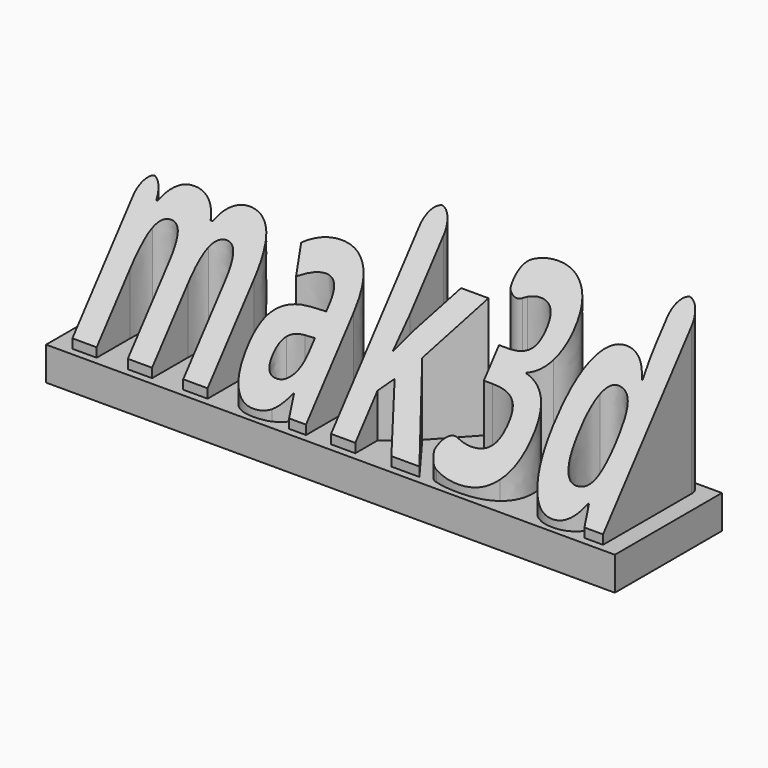
from build123d import *

# Parameters (mm, degrees)
F0_W         = 100
F0_H         = 20
F1_DEPTH     = 30
F4_DEPTH     = 15
F3_W         = 100
F3_H         = 20
F5_DEPTH     = 25
F6_DEPTH     = 200
F7_T4_DEPTH  = 29.5243209298
F7_T9_DEPTH  = 29.5243209298
F7_T14_DEPTH = 29.5243209298
F7_T19_DEPTH = 29.5243209298
F7_T24_DEPTH = 23.0076746252
F7_T29_DEPTH = 21.7768646713
F7_T34_DEPTH = 22.6661302513
F7_T39_DEPTH = 27.5964135534
F7_T44_DEPTH = 6.1840354013
F7_T49_DEPTH = 13.2594596433


# Not quite as in the source:
# - a fillet or chamfer that OpenCascade refuses, or shapes differently, is made with other operations: its cross-section is extruded or revolved along the edge and cut away or added


with BuildPart() as f1:
    # F0 (on Top) → F1 (new body)
    with BuildSketch(Plane.XY):
        with Locations((-50, 10)):
            Rectangle(F0_W, F0_H)
    extrude(amount=F1_DEPTH)

    # F4 (cut): a face of the model
    f4_faces = [f1.faces().sort_by_distance(p)[0] for p in [
        (0, 10, 15),
    ]]
    extrude(f4_faces, amount=-F4_DEPTH, mode=Mode.SUBTRACT)

    # F3 (on face) → F5 (cut)
    with BuildSketch(Plane.XY.offset(30)):
        with Locations((-50, 10)):
            Rectangle(F3_W, F3_H)
        with BuildLine():
            Line((-85.037182828, 7.7762018089), (-85.037182828, 1.100566471))
            Line((-85.037182828, 1.100566471), (-88.6663217196, 1.100566471))
            Line((-88.6663217196, 1.100566471), (-88.6663217196, 8.8729405296))
            add(Edge.make_bspline(
                [(-88.6663217196, 8.8729405296), (-88.6663217196, 10.3124101004), (-89.1480489702, 11.0321448859)],
                knots=[0, 0, 0, 1, 1, 1], degree=2))
            add(Edge.make_bspline(
                [(-89.1480489702, 11.0321448859), (-89.6297762207, 11.7518796713), (-90.6655850125, 11.7518796713)],
                knots=[0, 0, 0, 1, 1, 1], degree=2))
            add(Edge.make_bspline(
                [(-90.6655850125, 11.7518796713), (-92.0593571367, 11.7518796713), (-92.689601089, 10.7274952413)],
                knots=[0, 0, 0, 1, 1, 1], degree=2))
            add(Edge.make_bspline(
                [(-92.689601089, 10.7274952413), (-93.3198450413, 9.7031108112), (-93.3198450413, 7.3611166681)],
                knots=[0, 0, 0, 1, 1, 1], degree=2))
            Line((-93.3198450413, 7.3611166681), (-93.3198450413, 1.100566471))
            Line((-93.3198450413, 1.100566471), (-96.9489839329, 1.100566471))
            Line((-96.9489839329, 1.100566471), (-96.9489839329, 14.4061397001))
            Line((-96.9489839329, 14.4061397001), (-94.1766721668, 14.4061397001))
            Line((-94.1766721668, 14.4061397001), (-93.6892327354, 12.7039098108))
            Line((-93.6892327354, 12.7039098108), (-93.4874023458, 12.7039098108))
            add(Edge.make_bspline(
                [(-93.4874023458, 12.7039098108), (-92.9504573472, 13.6216668652), (-91.9394013391, 14.1376672008)],
                knots=[0, 0, 0, 1, 1, 1], degree=2))
            add(Edge.make_bspline(
                [(-91.9394013391, 14.1376672008), (-90.928345331, 14.6536675364), (-89.6183518591, 14.6536675364)],
                knots=[0, 0, 0, 1, 1, 1], degree=2))
            add(Edge.make_bspline(
                [(-89.6183518591, 14.6536675364), (-86.6327853417, 14.6536675364), (-85.5703197061, 12.7039098108)],
                knots=[0, 0, 0, 1, 1, 1], degree=2))
            Line((-85.5703197061, 12.7039098108), (-85.2504375792, 12.7039098108))
            add(Edge.make_bspline(
                [(-85.2504375792, 12.7039098108), (-84.7134925806, 13.6330912269), (-83.6738756683, 14.1433793816)],
                knots=[0, 0, 0, 1, 1, 1], degree=2))
            add(Edge.make_bspline(
                [(-83.6738756683, 14.1433793816), (-82.634258756, 14.6536675364), (-81.3242652841, 14.6536675364)],
                knots=[0, 0, 0, 1, 1, 1], degree=2))
            add(Edge.make_bspline(
                [(-81.3242652841, 14.6536675364), (-79.0622416727, 14.6536675364), (-77.9026689628, 13.4940948265)],
                knots=[0, 0, 0, 1, 1, 1], degree=2))
            add(Edge.make_bspline(
                [(-77.9026689628, 13.4940948265), (-76.743096253, 12.3345221167), (-76.743096253, 9.7754651018)],
                knots=[0, 0, 0, 1, 1, 1], degree=2))
            Line((-76.743096253, 9.7754651018), (-76.743096253, 1.100566471))
            Line((-76.743096253, 1.100566471), (-80.3836595063, 1.100566471))
            Line((-80.3836595063, 1.100566471), (-80.3836595063, 8.8729405296))
            add(Edge.make_bspline(
                [(-80.3836595063, 8.8729405296), (-80.3836595063, 10.3124101004), (-80.8653867568, 11.0321448859)],
                knots=[0, 0, 0, 1, 1, 1], degree=2))
            add(Edge.make_bspline(
                [(-80.8653867568, 11.0321448859), (-81.3471140074, 11.7518796713), (-82.3829227991, 11.7518796713)],
                knots=[0, 0, 0, 1, 1, 1], degree=2))
            add(Edge.make_bspline(
                [(-82.3829227991, 11.7518796713), (-83.7157649944, 11.7518796713), (-84.3764739112, 10.7998495318)],
                knots=[0, 0, 0, 1, 1, 1], degree=2))
            add(Edge.make_bspline(
                [(-84.3764739112, 10.7998495318), (-85.037182828, 9.8478193924), (-85.037182828, 7.7762018089)],
                knots=[0, 0, 0, 1, 1, 1], degree=2))
        make_face(mode=Mode.SUBTRACT)
        with BuildLine():
            Line((-62.0361346585, 1.100566471), (-64.5685348295, 1.100566471))
            Line((-64.5685348295, 1.100566471), (-65.2730371327, 2.909423736))
            Line((-65.2730371327, 2.909423736), (-65.3682401467, 2.909423736))
            add(Edge.make_bspline(
                [(-65.3682401467, 2.909423736), (-66.2821890805, 1.7555632069), (-67.2532598228, 1.3081090414)],
                knots=[0, 0, 0, 1, 1, 1], degree=2))
            add(Edge.make_bspline(
                [(-67.2532598228, 1.3081090414), (-68.224330565, 0.8606548759), (-69.7818518732, 0.8606548759)],
                knots=[0, 0, 0, 1, 1, 1], degree=2))
            add(Edge.make_bspline(
                [(-69.7818518732, 0.8606548759), (-71.6973365138, 0.8606548759), (-72.797883355, 1.9573935965)],
                knots=[0, 0, 0, 1, 1, 1], degree=2))
            add(Edge.make_bspline(
                [(-72.797883355, 1.9573935965), (-73.8984301962, 3.0541323172), (-73.8984301962, 5.0762443334)],
                knots=[0, 0, 0, 1, 1, 1], degree=2))
            add(Edge.make_bspline(
                [(-73.8984301962, 5.0762443334), (-73.8984301962, 7.1935593636), (-72.4170712992, 8.1989031908)],
                knots=[0, 0, 0, 1, 1, 1], degree=2))
            add(Edge.make_bspline(
                [(-72.4170712992, 8.1989031908), (-70.9357124022, 9.2042470181), (-67.9501458849, 9.3108743937)],
                knots=[0, 0, 0, 1, 1, 1], degree=2))
            Line((-67.9501458849, 9.3108743937), (-65.6386167063, 9.3832286843))
            Line((-65.6386167063, 9.3832286843), (-65.6386167063, 9.9658711297))
            add(Edge.make_bspline(
                [(-65.6386167063, 9.9658711297), (-65.6386167063, 11.9879831459), (-67.7102342897, 11.9879831459)],
                knots=[0, 0, 0, 1, 1, 1], degree=2))
            add(Edge.make_bspline(
                [(-67.7102342897, 11.9879831459), (-69.3058368035, 11.9879831459), (-71.4612330392, 11.0245286448)],
                knots=[0, 0, 0, 1, 1, 1], degree=2))
            Line((-71.4612330392, 11.0245286448), (-72.6607910149, 13.476958284))
            add(Edge.make_bspline(
                [(-72.6607910149, 13.476958284), (-70.3644943186, 14.6803243803), (-67.5693338291, 14.6803243803)],
                knots=[0, 0, 0, 1, 1, 1], degree=2))
            add(Edge.make_bspline(
                [(-67.5693338291, 14.6803243803), (-64.8922250769, 14.6803243803), (-63.4641798677, 13.5131354293)],
                knots=[0, 0, 0, 1, 1, 1], degree=2))
            add(Edge.make_bspline(
                [(-63.4641798677, 13.5131354293), (-62.0361346585, 12.3459464783), (-62.0361346585, 9.9658711297)],
                knots=[0, 0, 0, 1, 1, 1], degree=2))
            Line((-62.0361346585, 9.9658711297), (-62.0361346585, 1.100566471))
        make_face(mode=Mode.SUBTRACT)
        with BuildLine():
            add(Edge.make_bspline(
                [(-34.1911571395, 17.6525624757), (-32.6260195902, 16.5577278153), (-32.6260195902, 14.6079700897)],
                knots=[0, 0, 0, 1, 1, 1], degree=2))
            add(Edge.make_bspline(
                [(-32.6260195902, 14.6079700897), (-32.6260195902, 12.9780944909), (-33.614226875, 11.8356583236)],
                knots=[0, 0, 0, 1, 1, 1], degree=2))
            add(Edge.make_bspline(
                [(-33.614226875, 11.8356583236), (-34.6024341598, 10.6932221562), (-36.3884427014, 10.2629045332)],
                knots=[0, 0, 0, 1, 1, 1], degree=2))
            Line((-36.3884427014, 10.2629045332), (-36.3884427014, 10.1943583632))
            add(Edge.make_bspline(
                [(-36.3884427014, 10.1943583632), (-34.2787439123, 9.9315980447), (-33.1972376739, 8.9129257954)],
                knots=[0, 0, 0, 1, 1, 1], degree=2))
            add(Edge.make_bspline(
                [(-33.1972376739, 8.9129257954), (-32.1157314355, 7.8942535462), (-32.1157314355, 6.1691749335)],
                knots=[0, 0, 0, 1, 1, 1], degree=2))
            add(Edge.make_bspline(
                [(-32.1157314355, 6.1691749335), (-32.1157314355, 3.6596234859), (-33.9360130621, 2.2601391809)],
                knots=[0, 0, 0, 1, 1, 1], degree=2))
            add(Edge.make_bspline(
                [(-33.9360130621, 2.2601391809), (-35.7562946888, 0.8606548759), (-39.1340976236, 0.8606548759)],
                knots=[0, 0, 0, 1, 1, 1], degree=2))
            add(Edge.make_bspline(
                [(-39.1340976236, 0.8606548759), (-41.9673393186, 0.8606548759), (-44.1570086394, 1.8012606536)],
                knots=[0, 0, 0, 1, 1, 1], degree=2))
            Line((-44.1570086394, 1.8012606536), (-44.1570086394, 4.9315357522))
            add(Edge.make_bspline(
                [(-44.1570086394, 4.9315357522), (-43.1478566916, 4.4212475974), (-41.9330662336, 4.0994614103)],
                knots=[0, 0, 0, 1, 1, 1], degree=2))
            add(Edge.make_bspline(
                [(-41.9330662336, 4.0994614103), (-40.7182757757, 3.7776752232), (-39.5301421616, 3.7776752232)],
                knots=[0, 0, 0, 1, 1, 1], degree=2))
            add(Edge.make_bspline(
                [(-39.5301421616, 3.7776752232), (-37.7060524144, 3.7776752232), (-36.8378009272, 4.3964948138)],
                knots=[0, 0, 0, 1, 1, 1], degree=2))
            add(Edge.make_bspline(
                [(-36.8378009272, 4.3964948138), (-35.96954944, 5.0153144045), (-35.96954944, 6.3862378053)],
                knots=[0, 0, 0, 1, 1, 1], degree=2))
            add(Edge.make_bspline(
                [(-35.96954944, 6.3862378053), (-35.96954944, 7.6086445044), (-36.9691810865, 8.1208367194)],
                knots=[0, 0, 0, 1, 1, 1], degree=2))
            add(Edge.make_bspline(
                [(-36.9691810865, 8.1208367194), (-37.9688127329, 8.6330289344), (-40.1584820537, 8.6330289344)],
                knots=[0, 0, 0, 1, 1, 1], degree=2))
            Line((-40.1584820537, 8.6330289344), (-41.4798998872, 8.6330289344))
            Line((-41.4798998872, 8.6330289344), (-41.4798998872, 11.4548462678))
            Line((-41.4798998872, 11.4548462678), (-40.1356333303, 11.4548462678))
            add(Edge.make_bspline(
                [(-40.1356333303, 11.4548462678), (-38.1135213141, 11.4548462678), (-37.1786277171, 11.9841750253)],
                knots=[0, 0, 0, 1, 1, 1], degree=2))
            add(Edge.make_bspline(
                [(-37.1786277171, 11.9841750253), (-36.2437341202, 12.5135037829), (-36.2437341202, 13.7968404109)],
                knots=[0, 0, 0, 1, 1, 1], degree=2))
            add(Edge.make_bspline(
                [(-36.2437341202, 13.7968404109), (-36.2437341202, 15.7732549804), (-38.7190124828, 15.7732549804)],
                knots=[0, 0, 0, 1, 1, 1], degree=2))
            add(Edge.make_bspline(
                [(-38.7190124828, 15.7732549804), (-39.5758396083, 15.7732549804), (-40.4631316983, 15.4876459386)],
                knots=[0, 0, 0, 1, 1, 1], degree=2))
            add(Edge.make_bspline(
                [(-40.4631316983, 15.4876459386), (-41.3504237883, 15.2020368967), (-42.4319300267, 14.5013427141)],
                knots=[0, 0, 0, 1, 1, 1], degree=2))
            Line((-42.4319300267, 14.5013427141), (-44.1341599161, 17.0337428851))
            add(Edge.make_bspline(
                [(-44.1341599161, 17.0337428851), (-41.7540845674, 18.7473971361), (-38.4562521643, 18.7473971361)],
                knots=[0, 0, 0, 1, 1, 1], degree=2))
            add(Edge.make_bspline(
                [(-38.4562521643, 18.7473971361), (-35.7562946888, 18.7473971361), (-34.1911571395, 17.6525624757)],
                knots=[0, 0, 0, 1, 1, 1], degree=2))
        make_face(mode=Mode.SUBTRACT)
        Polygon((-54.857827407, 8.3359955309), (-54.8083218397, 8.3359955309), (-53.2279518082, 10.3581075471), (-49.5036099026, 14.4061397001), (-45.4098803029, 14.4061397001), (-50.6917435167, 8.6330289344), (-45.0861900555, 1.100566471), (-49.2751226692, 1.100566471), (-53.1060919504, 6.4928651809), (-54.6674213791, 5.2438016379), (-54.6674213791, 1.100566471), (-58.2965602707, 1.100566471), (-58.2965602707, 19.6194567438), (-54.6674213791, 19.6194567438), (-54.6674213791, 11.3596432539), align=None, mode=Mode.SUBTRACT)
        with BuildLine():
            add(Edge.make_bspline(
                [(-21.2854365689, 2.8256450837), (-22.5230757502, 0.8606548759), (-25.0592840418, 0.8606548759)],
                knots=[0, 0, 0, 1, 1, 1], degree=2))
            add(Edge.make_bspline(
                [(-25.0592840418, 0.8606548759), (-27.4012781848, 0.8606548759), (-28.7398325609, 2.6828405628)],
                knots=[0, 0, 0, 1, 1, 1], degree=2))
            add(Edge.make_bspline(
                [(-28.7398325609, 2.6828405628), (-30.078386937, 4.5050262497), (-30.078386937, 7.7305043622)],
                knots=[0, 0, 0, 1, 1, 1], degree=2))
            add(Edge.make_bspline(
                [(-30.078386937, 7.7305043622), (-30.078386937, 11.0016799214), (-28.7169838376, 12.8276737289)],
                knots=[0, 0, 0, 1, 1, 1], degree=2))
            add(Edge.make_bspline(
                [(-28.7169838376, 12.8276737289), (-27.3555807382, 14.6536675364), (-24.9640810278, 14.6536675364)],
                knots=[0, 0, 0, 1, 1, 1], degree=2))
            add(Edge.make_bspline(
                [(-24.9640810278, 14.6536675364), (-22.4507214596, 14.6536675364), (-21.1293036261, 12.7039098108)],
                knots=[0, 0, 0, 1, 1, 1], degree=2))
            Line((-21.1293036261, 12.7039098108), (-21.0112518888, 12.7039098108))
            add(Edge.make_bspline(
                [(-21.0112518888, 12.7039098108), (-21.2854365689, 14.1928849489), (-21.2854365689, 15.3581698396)],
                knots=[0, 0, 0, 1, 1, 1], degree=2))
            Line((-21.2854365689, 15.3581698396), (-21.2854365689, 19.6194567438))
            Line((-21.2854365689, 19.6194567438), (-17.6448733156, 19.6194567438))
            Line((-17.6448733156, 19.6194567438), (-17.6448733156, 1.100566471))
            Line((-17.6448733156, 1.100566471), (-20.4286094434, 1.100566471))
            Line((-20.4286094434, 1.100566471), (-21.1293036261, 2.8256450837))
            Line((-21.1293036261, 2.8256450837), (-21.2854365689, 2.8256450837))
        make_face(mode=Mode.SUBTRACT)
        with BuildLine():
            Line((-65.6386167063, 6.1691749335), (-65.6386167063, 7.2659136542))
            Line((-65.6386167063, 7.2659136542), (-67.0438131921, 7.2164080869))
            add(Edge.make_bspline(
                [(-67.0438131921, 7.2164080869), (-68.6279913442, 7.1707106402), (-69.4010398174, 6.6470940635)],
                knots=[0, 0, 0, 1, 1, 1], degree=2))
            add(Edge.make_bspline(
                [(-69.4010398174, 6.6470940635), (-70.1740882907, 6.1234774868), (-70.1740882907, 5.05339561)],
                knots=[0, 0, 0, 1, 1, 1], degree=2))
            add(Edge.make_bspline(
                [(-70.1740882907, 5.05339561), (-70.1740882907, 3.5149149047), (-68.4147365929, 3.5149149047)],
                knots=[0, 0, 0, 1, 1, 1], degree=2))
            add(Edge.make_bspline(
                [(-68.4147365929, 3.5149149047), (-67.1504405677, 3.5149149047), (-66.394528637, 4.2422659312)],
                knots=[0, 0, 0, 1, 1, 1], degree=2))
            add(Edge.make_bspline(
                [(-66.394528637, 4.2422659312), (-65.6386167063, 4.9696169578), (-65.6386167063, 6.1691749335)],
                knots=[0, 0, 0, 1, 1, 1], degree=2))
        make_face()
        with BuildLine():
            add(Edge.make_bspline(
                [(-25.7257051394, 4.7373216037), (-25.0478596801, 3.7548264998), (-23.7835636549, 3.7548264998)],
                knots=[0, 0, 0, 1, 1, 1], degree=2))
            add(Edge.make_bspline(
                [(-23.7835636549, 3.7548264998), (-22.3935996513, 3.7548264998), (-21.7443150962, 4.5640521184)],
                knots=[0, 0, 0, 1, 1, 1], degree=2))
            add(Edge.make_bspline(
                [(-21.7443150962, 4.5640521184), (-21.095030541, 5.3732777369), (-21.0341006121, 7.3116111009)],
                knots=[0, 0, 0, 1, 1, 1], degree=2))
            Line((-21.0341006121, 7.3116111009), (-21.0341006121, 7.7038475183))
            add(Edge.make_bspline(
                [(-21.0341006121, 7.7038475183), (-21.0341006121, 9.8478193924), (-21.6948095289, 10.7750967482)],
                knots=[0, 0, 0, 1, 1, 1], degree=2))
            add(Edge.make_bspline(
                [(-21.6948095289, 10.7750967482), (-22.3555184457, 11.7023741041), (-23.8444935838, 11.7023741041)],
                knots=[0, 0, 0, 1, 1, 1], degree=2))
            add(Edge.make_bspline(
                [(-23.8444935838, 11.7023741041), (-25.0592840418, 11.7023741041), (-25.7314173202, 10.6741815534)],
                knots=[0, 0, 0, 1, 1, 1], degree=2))
            add(Edge.make_bspline(
                [(-25.7314173202, 10.6741815534), (-26.4035505987, 9.6459890028), (-26.4035505987, 7.680998795)],
                knots=[0, 0, 0, 1, 1, 1], degree=2))
            add(Edge.make_bspline(
                [(-26.4035505987, 7.680998795), (-26.4035505987, 5.7198167077), (-25.7257051394, 4.7373216037)],
                knots=[0, 0, 0, 1, 1, 1], degree=2))
        make_face()
    extrude(amount=-F5_DEPTH, mode=Mode.SUBTRACT)

    # F2 (on face) → F6 (cut)
    with BuildSketch(Plane(origin=(-100, 0, 0), x_dir=(0, -1, 0), z_dir=(-1, 0, 0))):
        Polygon((-20, 30), (0, 5), (0, 30), align=None)
    extrude(amount=-F6_DEPTH, mode=Mode.SUBTRACT)

    # F7: fillet of radius 2 on 10 edges, made by hand


with BuildPart() as f7_tool2:
    # F7_s3 → F7_t4 (new body)
    with BuildSketch(Plane.XY.offset(34.5243209298)):
        with BuildLine():
            ThreePointArc((-17.6448733156, 17.6194567438), (-18.2306597533, 19.0336703062), (-19.6448733156, 19.6194567438))
            Line((-19.6448733156, 19.6194567438), (-19.6448733156, 19.6594567438))
            Line((-19.6448733156, 19.6594567438), (-17.6048733156, 19.6594567438))
            Line((-17.6048733156, 19.6594567438), (-17.6048733156, 17.6194567438))
            Line((-17.6048733156, 17.6194567438), (-17.6448733156, 17.6194567438))
        make_face()
    extrude(amount=-F7_T4_DEPTH)

    split(bisect_by=Plane(origin=(0, -2.4390243902, 1.9512195122), x_dir=(1, 0, 0), z_dir=(0, 0.7808688094, -0.6246950476)), keep=Keep.TOP)


with BuildPart() as f1_1:
    add(f1.part)

    # F7_t1: cut F7_tool2
    add(f7_tool2.part, mode=Mode.SUBTRACT)


with BuildPart() as f7_tool7:
    # F7_s8 → F7_t9 (new body)
    with BuildSketch(Plane.XY.offset(34.5243209298)):
        with BuildLine():
            ThreePointArc((-21.2854365689, 17.6194567438), (-20.6996501313, 19.0336703062), (-19.2854365689, 19.6194567438))
            Line((-19.2854365689, 19.6194567438), (-19.2854365689, 19.6594567438))
            Line((-19.2854365689, 19.6594567438), (-21.3254365689, 19.6594567438))
            Line((-21.3254365689, 19.6594567438), (-21.3254365689, 17.6194567438))
            Line((-21.3254365689, 17.6194567438), (-21.2854365689, 17.6194567438))
        make_face()
    extrude(amount=-F7_T9_DEPTH)

    split(bisect_by=Plane(origin=(0, -2.4390243902, 1.9512195122), x_dir=(1, 0, 0), z_dir=(0, 0.7808688094, -0.6246950476)), keep=Keep.TOP)


with BuildPart() as f1_2:
    add(f1_1.part)

    # F7_t6: cut F7_tool7
    add(f7_tool7.part, mode=Mode.SUBTRACT)


with BuildPart() as f7_tool12:
    # F7_s13 → F7_t14 (new body)
    with BuildSketch(Plane.XY.offset(34.5243209298)):
        with BuildLine():
            ThreePointArc((-56.2965602707, 19.6194567438), (-57.7107738331, 19.0336703062), (-58.2965602707, 17.6194567438))
            Line((-58.2965602707, 17.6194567438), (-58.3365602707, 17.6194567438))
            Line((-58.3365602707, 17.6194567438), (-58.3365602707, 19.6594567438))
            Line((-58.3365602707, 19.6594567438), (-56.2965602707, 19.6594567438))
            Line((-56.2965602707, 19.6594567438), (-56.2965602707, 19.6194567438))
        make_face()
    extrude(amount=-F7_T14_DEPTH)

    split(bisect_by=Plane(origin=(0, -2.4390243902, 1.9512195122), x_dir=(1, 0, 0), z_dir=(0, 0.7808688094, -0.6246950476)), keep=Keep.TOP)


with BuildPart() as f1_3:
    add(f1_2.part)

    # F7_t11: cut F7_tool12
    add(f7_tool12.part, mode=Mode.SUBTRACT)


with BuildPart() as f7_tool17:
    # F7_s18 → F7_t19 (new body)
    with BuildSketch(Plane.XY.offset(34.5243209298)):
        with BuildLine():
            ThreePointArc((-54.6674213791, 17.6194567438), (-55.2532078167, 19.0336703062), (-56.6674213791, 19.6194567438))
            Line((-56.6674213791, 19.6194567438), (-56.6674213791, 19.6594567438))
            Line((-56.6674213791, 19.6594567438), (-54.6274213791, 19.6594567438))
            Line((-54.6274213791, 19.6594567438), (-54.6274213791, 17.6194567438))
            Line((-54.6274213791, 17.6194567438), (-54.6674213791, 17.6194567438))
        make_face()
    extrude(amount=-F7_T19_DEPTH)

    split(bisect_by=Plane(origin=(0, -2.4390243902, 1.9512195122), x_dir=(1, 0, 0), z_dir=(0, 0.7808688094, -0.6246950476)), keep=Keep.TOP)


with BuildPart() as f1_4:
    add(f1_3.part)

    # F7_t16: cut F7_tool17
    add(f7_tool17.part, mode=Mode.SUBTRACT)


with BuildPart() as f7_tool22:
    # F7_s23 → F7_t24 (new body)
    with BuildSketch(Plane.XY.offset(28.0076746252)):
        with BuildLine():
            ThreePointArc((-96.9489839329, 12.4061397001), (-96.3631974953, 13.8203532625), (-94.9489839329, 14.4061397001))
            Line((-94.9489839329, 14.4061397001), (-94.9489839329, 14.4461397001))
            Line((-94.9489839329, 14.4461397001), (-96.9889839329, 14.4461397001))
            Line((-96.9889839329, 14.4461397001), (-96.9889839329, 12.4061397001))
            Line((-96.9889839329, 12.4061397001), (-96.9489839329, 12.4061397001))
        make_face()
    extrude(amount=-F7_T24_DEPTH)

    split(bisect_by=Plane(origin=(0, -2.4390243902, 1.9512195122), x_dir=(1, 0, 0), z_dir=(0, 0.7808688094, -0.6246950476)), keep=Keep.TOP)


with BuildPart() as f1_5:
    add(f1_4.part)

    # F7_t21: cut F7_tool22
    add(f7_tool22.part, mode=Mode.SUBTRACT)


with BuildPart() as f7_tool27:
    # F7_s28 → F7_t29 (new body)
    with BuildSketch(Plane.XY.offset(26.7768646713)):
        with BuildLine():
            ThreePointArc((-95.6843481853, 14.4061397001), (-94.4804289094, 14.003192729), (-93.7616252591, 12.9567180772))
            Line((-93.7616252591, 12.9567180772), (-93.7231708006, 12.9677296447))
            Line((-93.7231708006, 12.9677296447), (-94.1465186465, 14.4461397001))
            Line((-94.1465186465, 14.4461397001), (-95.6843481853, 14.4461397001))
            Line((-95.6843481853, 14.4461397001), (-95.6843481853, 14.4061397001))
        make_face()
    extrude(amount=-F7_T29_DEPTH)

    split(bisect_by=Plane(origin=(0, -2.4390243902, 1.9512195122), x_dir=(1, 0, 0), z_dir=(0, 0.7808688094, -0.6246950476)), keep=Keep.TOP)


with BuildPart() as f1_6:
    add(f1_5.part)

    # F7_t26: cut F7_tool27
    add(f7_tool27.part, mode=Mode.SUBTRACT)


with BuildPart() as f7_tool32:
    # F7_s33 → F7_t34 (new body)
    with BuildSketch(Plane.XY.offset(27.6661302513)):
        with BuildLine():
            ThreePointArc((-43.4448891387, 16.0083176793), (-42.3498554722, 15.2054617052), (-40.9944804964, 15.2869179565))
            Line((-40.9944804964, 15.2869179565), (-40.9786696128, 15.2501753931))
            ThreePointArc((-40.9786696128, 15.2501753931), (-41.7103205764, 14.8889104737), (-42.4101803746, 14.4677725989))
            Line((-42.4101803746, 14.4677725989), (-42.465127316, 14.4790281452))
            Line((-42.465127316, 14.4790281452), (-43.4780864279, 15.9860031104))
            Line((-43.4780864279, 15.9860031104), (-43.4448891387, 16.0083176793))
        make_face()
    extrude(amount=-F7_T34_DEPTH)

    split(bisect_by=Plane(origin=(0, -2.4390243902, 1.9512195122), x_dir=(1, 0, 0), z_dir=(0, 0.7808688094, -0.6246950476)), keep=Keep.TOP)


with BuildPart() as f1_7:
    add(f1_6.part)

    # F7_t31: cut F7_tool32
    add(f7_tool32.part, mode=Mode.SUBTRACT)


with BuildPart() as f7_tool37:
    # F7_s38 → F7_t39 (new body)
    with BuildSketch(Plane.XY.offset(32.5964135534)):
        with BuildLine():
            ThreePointArc((-41.8972083643, 18.1977825225), (-43.1351774331, 16.9415628517), (-42.8974857117, 15.1939479278))
            Line((-42.8974857117, 15.1939479278), (-42.930683001, 15.1716333589))
            Line((-42.930683001, 15.1716333589), (-44.1673572053, 17.0114283162))
            Line((-44.1673572053, 17.0114283162), (-44.1575321051, 17.0662042587))
            ThreePointArc((-44.1575321051, 17.0662042587), (-43.0763220048, 17.7323272545), (-41.9104001066, 18.2355446456))
            Line((-41.9104001066, 18.2355446456), (-41.8972083643, 18.1977825225))
        make_face()
    extrude(amount=-F7_T39_DEPTH)

    split(bisect_by=Plane(origin=(0, -2.4390243902, 1.9512195122), x_dir=(1, 0, 0), z_dir=(0, 0.7808688094, -0.6246950476)), keep=Keep.TOP)


with BuildPart() as f1_8:
    add(f1_7.part)

    # F7_t36: cut F7_tool37
    add(f7_tool37.part, mode=Mode.SUBTRACT)


with BuildPart() as f7_tool42:
    # F7_s43 → F7_t44 (new body)
    with BuildSketch(Plane.XY.offset(11.1840354013)):
        with BuildLine():
            ThreePointArc((-42.6693687447, 1.2901777986), (-43.7420512588, 2.0037475194), (-44.1570086394, 3.223435961))
            Line((-44.1570086394, 3.223435961), (-44.1970086394, 3.223435961))
            Line((-44.1970086394, 3.223435961), (-44.1970086394, 1.8012606536))
            Line((-44.1970086394, 1.8012606536), (-44.1727962625, 1.7645080897))
            ThreePointArc((-44.1727962625, 1.7645080897), (-43.4355182873, 1.4805650976), (-42.6796159468, 1.2515126354))
            Line((-42.6796159468, 1.2515126354), (-42.6693687447, 1.2901777986))
        make_face()
    extrude(amount=-F7_T44_DEPTH)

    split(bisect_by=Plane(origin=(0, -2.4390243902, 1.9512195122), x_dir=(1, 0, 0), z_dir=(0, 0.7808688094, -0.6246950476)), keep=Keep.TOP)


with BuildPart() as f1_9:
    add(f1_8.part)

    # F7_t41: cut F7_tool42
    add(f7_tool42.part, mode=Mode.SUBTRACT)


with BuildPart() as f7_tool47:
    # F7_s48 → F7_t49 (new body)
    with BuildSketch(Plane.XY.offset(18.2594596433)):
        with BuildLine():
            ThreePointArc((-44.1570086394, 2.093519771), (-43.3959287607, 3.6635761181), (-41.6919317063, 4.0386941709))
            Line((-41.6919317063, 4.0386941709), (-41.6826301676, 4.0775976589))
            ThreePointArc((-41.6826301676, 4.0775976589), (-42.9362472843, 4.4522804058), (-44.1389586363, 4.9672316538))
            Line((-44.1389586363, 4.9672316538), (-44.1970086394, 4.9315357522))
            Line((-44.1970086394, 4.9315357522), (-44.1970086394, 2.093519771))
            Line((-44.1970086394, 2.093519771), (-44.1570086394, 2.093519771))
        make_face()
    extrude(amount=-F7_T49_DEPTH)

    split(bisect_by=Plane(origin=(0, -2.4390243902, 1.9512195122), x_dir=(1, 0, 0), z_dir=(0, 0.7808688094, -0.6246950476)), keep=Keep.TOP)


with BuildPart() as f1_10:
    add(f1_9.part)

    # F7_t46: cut F7_tool47
    add(f7_tool47.part, mode=Mode.SUBTRACT)


solid = f1_10.part
